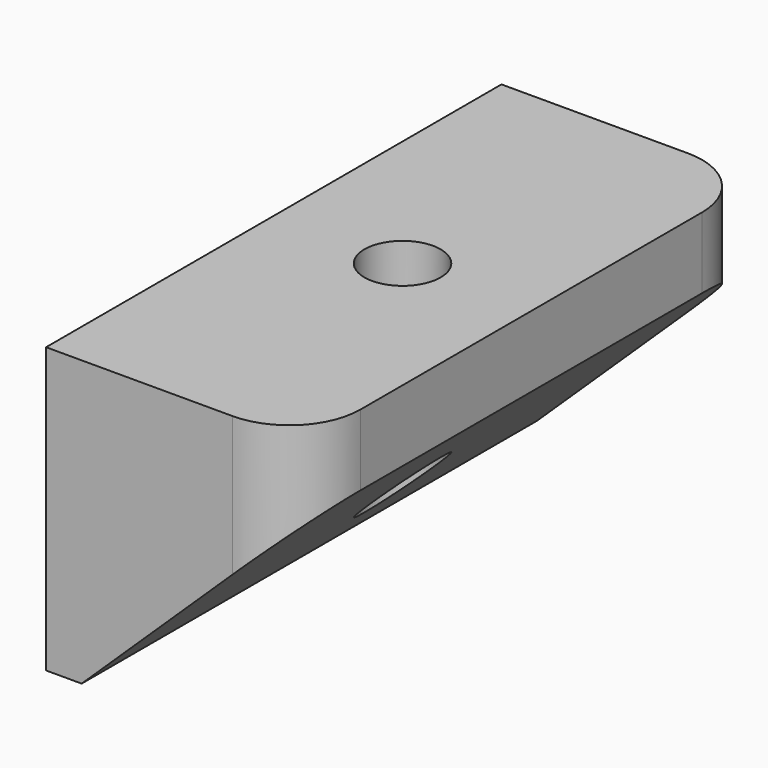
from build123d import *

# Parameters (mm, degrees)
F0_W        = 22.987
F0_H        = 25.4
F1_DEPTH    = 25.4
F2_R        = 6.35
F4_D        = 6.8
F5_T1_DEPTH = 140.0532259942


# Not quite as in the source:
# - a fillet or chamfer that OpenCascade refuses, or shapes differently, is made with other operations: its cross-section is extruded or revolved along the edge and cut away or added


with BuildPart() as f1:
    # F0 (on Front) → F1 (new body, symmetric)
    with BuildSketch(Plane.XZ):
        Rectangle(F0_W, F0_H)
    extrude(amount=F1_DEPTH, both=True)

    # F2
    f2_edges = [f1.edges().sort_by_distance(p)[0] for p in [
        (11.4935, 25.4, 0),
        (11.4935, -25.4, 0),
    ]]
    fillet(f2_edges, radius=F2_R)

    # F4 (through all)
    with Locations(Plane.XY.offset(12.7)):
        with Locations((0, 0)):
            Hole(F4_D / 2)

    # F5: chamfer of 19.05 x 19.812 on 1 edges, made by hand

    # F5_s2 → F5_t1 (cut)
    with BuildSketch(Plane.XZ.offset(-70.0266129971)):
        Polygon((11.4935, 6.35), (-8.3185, -12.7), (11.4935, -12.7), align=None)
    extrude(amount=F5_T1_DEPTH, mode=Mode.SUBTRACT)


solid = f1.part
